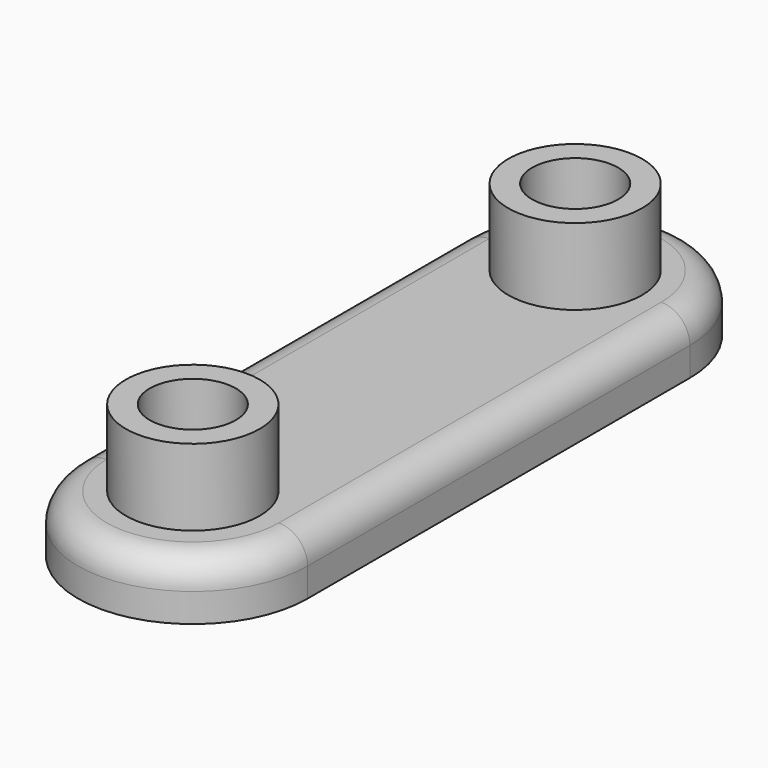
from build123d import *

# Parameters (mm, degrees)
F1_DEPTH       = 3
F2_R           = 3.5
F3_DEPTH       = 4
F5_D           = 4.5
F5_CSINK_D     = 9
F5_CSINK_ANGLE = 90
F6_R           = 1.5


# Not quite as in the source:
# - a feature names something its author has since deleted; it is built from what else it names


with BuildPart() as f1:
    # F0 (on Top) → F1 (new body)
    with BuildSketch(Plane.XY):
        with BuildLine():
            ThreePointArc((6, 12.5), (0, 18.5), (-6, 12.5))
            Line((-6, 12.5), (-6, -12.5))
            ThreePointArc((-6, -12.5), (0, -18.5), (6, -12.5))
            Line((6, -12.5), (6, 12.5))
        make_face()
    extrude(amount=F1_DEPTH)

    # F2 (on face) → F3 (join)
    with BuildSketch(Plane.XY.offset(3)):
        with Locations((0, -12.5)):
            Circle(F2_R)
        with Locations((0, 12.5)):
            Circle(F2_R)
    extrude(amount=F3_DEPTH)

    # F5 (through all)
    with Locations(Plane(origin=(0, 0, 0), x_dir=(1, 0, 0), z_dir=(0, 0, -1))):
        with Locations((0, 12.5), (0, -12.5)):
            CounterSinkHole(F5_D / 2, F5_CSINK_D / 2, counter_sink_angle=F5_CSINK_ANGLE)

    # F6
    f6_edges = [f1.edges().sort_by_distance(p)[0] for p in [
        (-6, 0, 3),
    ]]
    fillet(f6_edges, radius=F6_R)


solid = f1.part
